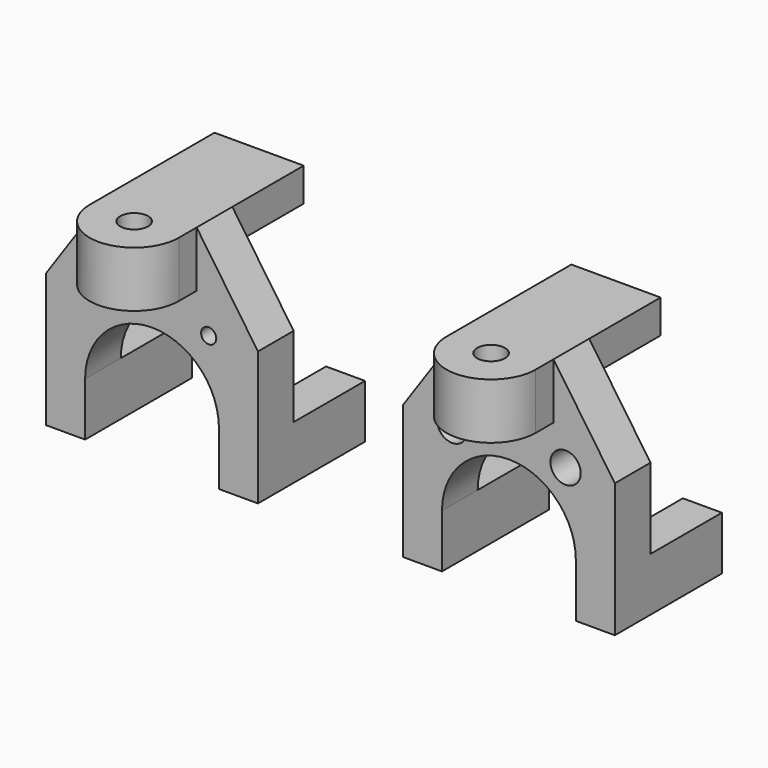
from build123d import *

# Parameters (mm, degrees)
F0_R      = 4.318
F1_DEPTH  = 12.7
F2_R      = 3.96875
F3_DEPTH  = 15.875
F4_W      = 25.4
F4_H      = 9.525
F4_W_2    = 11.1125
F4_H_2    = 15.24
F5_DEPTH  = 25.4
F7_R      = 4.318
F8_DEPTH  = 12.7
F9_R      = 2.159
F10_DEPTH = 38.101


with BuildPart() as f1:
    # F0 (on Front) → F1 (new body)
    with BuildSketch(Plane.XZ):
        with BuildLine():
            Line((19.05, -31.75), (30.1625, -31.75))
            Line((30.1625, -31.75), (30.1625, 6.35))
            Line((30.1625, 6.35), (12.7, 31.75))
            Line((12.7, 31.75), (-12.7, 31.75))
            Line((-12.7, 31.75), (-30.1625, 6.35))
            Line((-30.1625, 6.35), (-30.1625, -31.75))
            Line((-30.1625, -31.75), (-19.05, -31.75))
            Line((-19.05, -31.75), (-19.05, -16.51))
            ThreePointArc((-19.05, -16.51), (0, 2.54), (19.05, -16.51))
            Line((19.05, -16.51), (19.05, -31.75))
        make_face()
        with Locations((-16.129, 5.715)):
            Circle(F0_R, mode=Mode.SUBTRACT)
        with Locations((16.129, 5.715)):
            Circle(F0_R, mode=Mode.SUBTRACT)
    extrude(amount=F1_DEPTH)

    # F2 (on face) → F3 (join)
    with BuildSketch(Plane.XY.offset(31.75)):
        with BuildLine():
            Line((-12.7, 0), (-12.7, -19.05))
            ThreePointArc((-12.7, -19.05), (0, -31.75), (12.7, -19.05))
            Line((12.7, -19.05), (12.7, 0))
            Line((12.7, 0), (-12.7, 0))
        make_face()
        with Locations((0, -19.05)):
            Circle(F2_R, mode=Mode.SUBTRACT)
    extrude(amount=-F3_DEPTH)

    # F4 (on face) → F5 (join)
    with BuildSketch(Plane(origin=(0, 0, 0), x_dir=(-1, 0, 0), z_dir=(0, 1, 0))):
        with Locations((0, 26.9875)):
            Rectangle(F4_W, F4_H)
        with Locations((-24.60625, -24.13)):
            Rectangle(F4_W_2, F4_H_2)
        with Locations((24.60625, -24.13)):
            Rectangle(F4_W_2, F4_H_2)
    extrude(amount=F5_DEPTH)


with BuildPart() as f6_1:
    # F6: copy of F1
    add(f1.part.moved(Location((101.6, 0, 0))))


with BuildPart() as f1_1:
    add(f1.part)

    # F7 (on face) → F8 (join, through all)
    with BuildSketch(Plane.XZ):
        with Locations((16.129, 5.715)):
            Circle(F7_R)
        with Locations((-16.129, 5.715)):
            Circle(F7_R)
    extrude(amount=F8_DEPTH)

    # F9 (on face) → F10 (cut, through all)
    with BuildSketch(Plane.XZ.offset(12.7)):
        with Locations((-16.129, 5.715)):
            Circle(F9_R)
        with Locations((16.129, 5.715)):
            Circle(F9_R)
    extrude(amount=-F10_DEPTH, mode=Mode.SUBTRACT)


solid = Compound([f6_1.part, f1_1.part])
